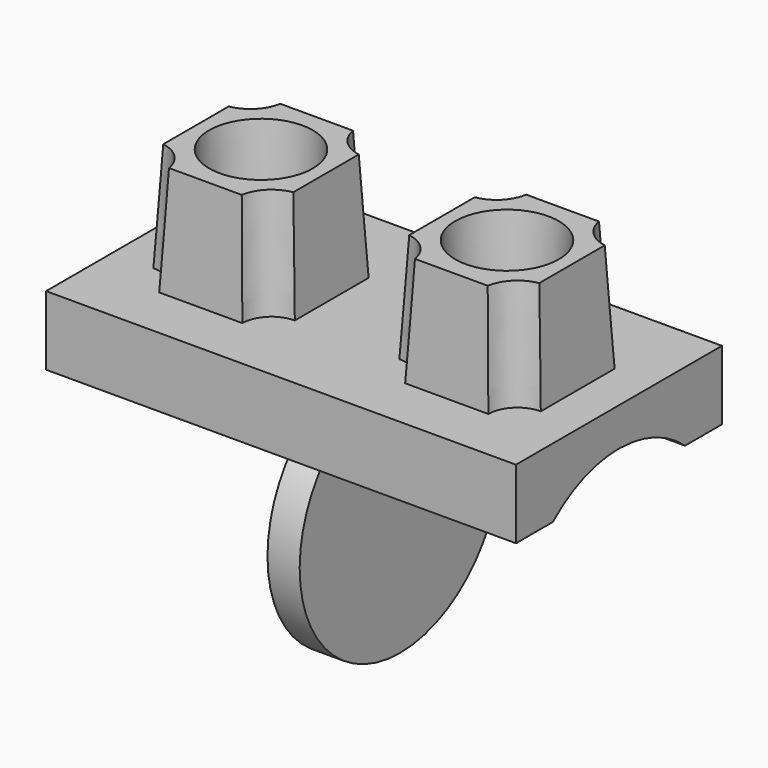
from build123d import *

# Parameters (mm, degrees)
F1_DEPTH               = 4
F2_R                   = 3.9
F3_DEPTH               = 7.301
F3_DEPTH_BACK          = 7.301
F4_DEPTH               = 0.5
F5_R                   = 1.431782869
F6_DEPTH               = 3.3837016672
DRAFT_F6_DRAFTED_ANGLE = 3


# Not quite as in the source:
# - an extrude with a draft is written as a straight extrude whose walls are then drafted


with BuildPart() as f1:
    # F0 (on Front) → F1 (new body, symmetric)
    with BuildSketch(Plane.XZ):
        Polygon((-7.3, 0), (7.3, 0), (7.3, 2.15), (0, 2.15), (-7.3, 2.15), align=None)
    extrude(amount=F1_DEPTH, both=True)

    # F2 (on Right) → F3 (cut, two sides)
    with BuildSketch(Plane.YZ) as f3_sk:
        with Locations((0, -2.9366769594)):
            Circle(F2_R)
    extrude(amount=-F3_DEPTH, mode=Mode.SUBTRACT)
    extrude(f3_sk.sketch, amount=F3_DEPTH_BACK, mode=Mode.SUBTRACT)

    # F2 (on Right) → F4 (join, symmetric)
    with BuildSketch(Plane.YZ):
        with Locations((0, -2.9366769594)):
            Circle(F2_R)
    extrude(amount=F4_DEPTH, both=True)


with BuildPart() as f6_drafted:
    # F5 (on face) → F6 (new body)
    with BuildSketch(Plane.XY.offset(2.15)):
        with BuildLine():
            ThreePointArc((-6.0191564262, -1.4343444008), (-5.3796870373, -1.6992212944), (-5.1148101437, -2.3386906832))
            Line((-5.1148101437, -2.3386906832), (-2.5284014893, -2.3386906832))
            ThreePointArc((-2.5284014893, -2.3386906832), (-2.2635245957, -1.6992212944), (-1.6240552068, -1.4343444008))
            Line((-1.6240552068, -1.4343444008), (-1.6240552068, 1.4343444008))
            ThreePointArc((-1.6240552068, 1.4343444008), (-2.2635245957, 1.6992212944), (-2.5284014893, 2.3386906832))
            Line((-2.5284014893, 2.3386906832), (-5.1148101437, 2.3386906832))
            ThreePointArc((-5.1148101437, 2.3386906832), (-5.3796870373, 1.6992212944), (-6.0191564262, 1.4343444008))
            Line((-6.0191564262, 1.4343444008), (-6.0191564262, -1.4343444008))
        make_face()
        with Locations((-3.8216058165, 0)):
            Circle(F5_R, mode=Mode.SUBTRACT)
    extrude(amount=F6_DEPTH)

    # draft_F6_drafted
    draft_f6_drafted_walls = [f6_drafted.faces().sort_by_distance(p)[0] for p in [
        (-6.0191564262, 0, 4.4058011115),
        (-5.3796870373, -1.6992212944, 4.4058011115),
        (-3.8216058165, -2.3386906832, 4.4058011115),
        (-2.2635245957, -1.6992212944, 4.4058011115),
        (-1.6240552068, 0, 4.4058011115),
        (-2.2635245957, 1.6992212944, 4.4058011115),
        (-3.8216058165, 2.3386906832, 4.4058011115),
        (-5.3796870373, 1.6992212944, 4.4058011115),
        (-5.2533886855, 0, 4.4058011115),
    ]]
    draft(draft_f6_drafted_walls, neutral_plane=Plane.XY.offset(2.15), angle=DRAFT_F6_DRAFTED_ANGLE)


with BuildPart() as f1_1:
    add(f1.part)

    # join_F6_drafted: union F6_drafted
    add(f6_drafted.part)

    # F7: F1 across plane


with BuildPart() as f1_2:
    add(f1_1.part)
    add(f1_1.part.mirror(Plane.YZ))


solid = f1_2.part
